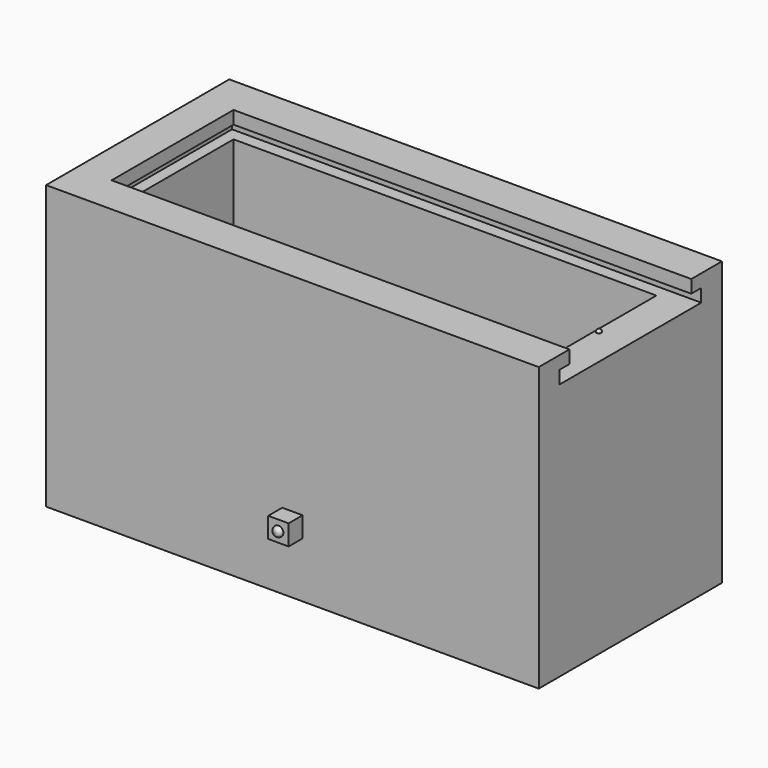
from build123d import *

# Parameters (mm, degrees)
F1_W      = 59.3920350075
F1_H      = 27.6011824608
F1_W_2    = 50.9779006243
F1_H_2    = 18.371000886
F2_DEPTH  = 25.4
F0_W      = 59.3920350075
F0_H      = 27.6011824608
F3_DEPTH  = 5.604719976
F18_DEPTH = 3.1209578738
F6_W      = 56.5673206002
F6_H      = 1.5604789369
F7_DEPTH  = 1.4987937175
F8_W      = 56.5673206002
F8_H      = 1.5604789369
F19_DEPTH = 1.4998847619
F5_W      = 21.3707275689
F5_H      = 1.5604789369
F9_DEPTH  = 1.382375136
F20_R     = 0.2935322564
F10_DEPTH = 0.3048
F21_R     = 0.254
F22_W     = 2.4601090699
F22_H     = 2.4032953017
F11_DEPTH = 2.1082
F12_R     = 0.5576398104
F13_DEPTH = 0.508
F14_R     = 0.50799
F23_W     = 2.4601090699
F23_H     = 2.4571502453
F15_DEPTH = 2.1082
F24_R     = 0.5965812211
F16_DEPTH = 0.508
F17_R     = 0.50799


# Not quite as in the source:
# - a fillet or chamfer is up to 0.001 mm smaller than in the source, because OpenCascade refuses the exact size


with BuildPart() as f2:
    # F1 (on face) → F2 (new body)
    with BuildSketch(Plane.XY):
        Rectangle(F1_W, F1_H)
        Rectangle(F1_W_2, F1_H_2, mode=Mode.SUBTRACT)
    extrude(amount=F2_DEPTH)

    # F0 (on Top) → F3 (join)
    with BuildSketch(Plane.XY):
        Rectangle(F0_W, F0_H)
    extrude(amount=-F3_DEPTH)

    # F4 (on face) → F18 (join)
    with BuildSketch(Plane.XY.offset(25.4)):
        Polygon((29.6960175037, -13.8005912304), (29.6960175037, -10.6853637844), (-26.8713030964, -10.6853637844), (-26.8713030964, 10.6853637844), (29.6960175037, 10.6853637844), (29.6960175037, 13.8005912304), (-29.6960175037, 13.8005912304), (-29.6960175037, -13.8005912304), align=None)
    extrude(amount=F18_DEPTH)

    # F6 (on face) → F7 (join)
    with BuildSketch(Plane.XZ.offset(-10.6853637844)):
        with Locations((1.4123572037, 27.7407184053)):
            Rectangle(F6_W, F6_H)
    extrude(amount=F7_DEPTH)

    # F8 (on face) → F19 (join)
    with BuildSketch(Plane(origin=(0, -10.6853637844, 0), x_dir=(-1, 0, 0), z_dir=(0, 1, 0))):
        with Locations((-1.4123572037, 27.7407184053)):
            Rectangle(F8_W, F8_H)
    extrude(amount=F19_DEPTH)

    # F5 (on face) → F9 (join)
    with BuildSketch(Plane.YZ.offset(-26.8713030964)):
        with Locations((0, 27.7407184053)):
            Rectangle(F5_W, F5_H)
    extrude(amount=F9_DEPTH)

    # F20 (on face) → F10 (join)
    with BuildSketch(Plane.XY.offset(25.4)):
        with Locations((25.8976798505, 0)):
            Circle(F20_R)
    extrude(amount=F10_DEPTH)

    # F21
    f21_edges = [f2.edges().sort_by_distance(p)[0] for p in [
        (25.604148, 0, 25.7048),
    ]]
    fillet(f21_edges, radius=F21_R)

    # F22 (on face) → F11 (join)
    with BuildSketch(Plane(origin=(0, 13.8005912304, 0), x_dir=(-1, 0, 0), z_dir=(0, 1, 0))):
        with Locations((0, 2.2958383197)):
            Rectangle(F22_W, F22_H)
    extrude(amount=F11_DEPTH)

    # F12 (on face) → F13 (join)
    with BuildSketch(Plane(origin=(0, 15.9087912304, 0), x_dir=(-1, 0, 0), z_dir=(0, 1, 0))):
        with Locations((0, 2.2958383197)):
            Circle(F12_R)
    extrude(amount=F13_DEPTH)

    # F14 (radius 0.508 in the source; OpenCascade refuses exactly that, so slightly less here)
    f14_edges = [f2.edges().sort_by_distance(p)[0] for p in [
        (0.55764, 16.416791, 2.295838),
    ]]
    fillet(f14_edges, radius=F14_R)

    # F23 (on face) → F15 (join)
    with BuildSketch(Plane.XZ.offset(13.8005912304)):
        with Locations((0, 2.3100455292)):
            Rectangle(F23_W, F23_H)
    extrude(amount=F15_DEPTH)

    # F24 (on face) → F16 (join)
    with BuildSketch(Plane.XZ.offset(15.9087912304)):
        with Locations((0, 2.3100455292)):
            Circle(F24_R)
    extrude(amount=F16_DEPTH)

    # F17 (radius 0.508 in the source; OpenCascade refuses exactly that, so slightly less here)
    f17_edges = [f2.edges().sort_by_distance(p)[0] for p in [
        (-0.596581, -16.416791, 2.310046),
    ]]
    fillet(f17_edges, radius=F17_R)


solid = f2.part
